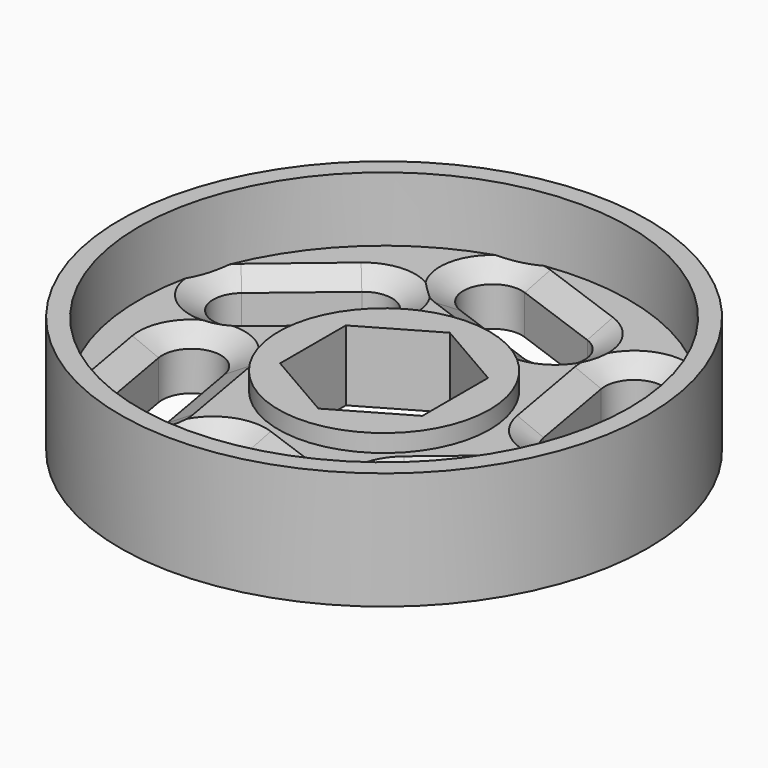
from build123d import *

# Parameters (mm, degrees)
F1_START     = 2
F0_R         = 20.9
F0_R_2       = 9
F1_DEPTH     = 4.5
F2_START     = 2
F0_R_3       = 8
F2_DEPTH     = 6
F3_START     = 2
F3_DEPTH     = 6
F4_START     = 2
F0_R_4       = 22.5
F4_DEPTH     = 10
F5_T1_DEPTH  = 8
F5_T3_DEPTH  = 8
F5_T5_DEPTH  = 8
F5_T7_DEPTH  = 8
F5_T9_DEPTH  = 8
F5_T11_DEPTH = 8
F5_T13_DEPTH = 8
F5_T15_DEPTH = 8
F5_T17_DEPTH = 8
F5_T19_DEPTH = 8
F5_T21_DEPTH = 8
F5_T23_DEPTH = 8
F5_T26_ANGLE = 180
F5_T30_ANGLE = 180
F5_S31_R     = 20.9
F5_T32_DEPTH = 7
F5_T34_ANGLE = 180
F5_T38_ANGLE = 180
F5_S39_R     = 20.9
F5_T40_DEPTH = 7
F5_T44_ANGLE = 180
F5_S45_R     = 20.9
F5_T46_DEPTH = 7
F5_T48_ANGLE = 180
F5_T52_ANGLE = 180
F5_S53_R     = 20.9
F5_T54_DEPTH = 7
F5_T56_ANGLE = 180
F5_T60_ANGLE = 180
F5_S61_R     = 20.9
F5_T62_DEPTH = 7
F5_T64_ANGLE = 180
F5_T66_ANGLE = 180
F5_T70_ANGLE = 180
F5_S71_R     = 20.9
F5_T72_DEPTH = 7


# Not quite as in the source:
# - a fillet or chamfer that OpenCascade refuses, or shapes differently, is made with other operations: its cross-section is extruded or revolved along the edge and cut away or added
# - a feature names something its author has since deleted; it is built from what else it names


with BuildPart() as f1:
    # F0 (on Top) → F1 (new body)
    with BuildSketch(Plane.XY.offset(F1_START)):
        Circle(F0_R)
        with BuildLine():
            ThreePointArc((4.6138208415, -13.9188490213), (6.1080020351, -17.1231309316), (2.9037201248, -18.6173121253))
            Line((2.9037201248, -18.6173121253), (-4.6138208415, -15.8811509787))
            ThreePointArc((-4.6138208415, -15.8811509787), (-6.1080020351, -12.6768690684), (-2.9037201248, -11.1826878747))
            Line((-2.9037201248, -11.1826878747), (4.6138208415, -13.9188490213))
        make_face(mode=Mode.SUBTRACT)
        with BuildLine():
            ThreePointArc((-9.7471664232, -10.9551105679), (-11.7750653616, -13.8512503946), (-14.6712051883, -11.8233514562))
            Line((-14.6712051883, -11.8233514562), (-16.0603906096, -3.9448894321))
            ThreePointArc((-16.0603906096, -3.9448894321), (-14.0324916712, -1.0487496054), (-11.1363518445, -3.0766485438))
            Line((-11.1363518445, -3.0766485438), (-9.7471664232, -10.9551105679))
        make_face(mode=Mode.SUBTRACT)
        with BuildLine():
            ThreePointArc((14.3609872646, -2.9637384535), (17.8830673967, -3.271880537), (17.5749253131, -6.7939606691))
            Line((17.5749253131, -6.7939606691), (11.4465697681, -11.9362615465))
            ThreePointArc((11.4465697681, -11.9362615465), (7.9244896361, -11.628119463), (8.2326317197, -8.1060393309))
            Line((8.2326317197, -8.1060393309), (14.3609872646, -2.9637384535))
        make_face(mode=Mode.SUBTRACT)
        with BuildLine():
            ThreePointArc((-14.3609872646, 2.9637384535), (-17.8830673967, 3.271880537), (-17.5749253131, 6.7939606691))
            Line((-17.5749253131, 6.7939606691), (-11.4465697681, 11.9362615465))
            ThreePointArc((-11.4465697681, 11.9362615465), (-7.9244896361, 11.628119463), (-8.2326317197, 8.1060393309))
            Line((-8.2326317197, 8.1060393309), (-14.3609872646, 2.9637384535))
        make_face(mode=Mode.SUBTRACT)
        Circle(F0_R_2, mode=Mode.SUBTRACT)
        with BuildLine():
            ThreePointArc((9.7471664232, 10.9551105679), (11.7750653616, 13.8512503946), (14.6712051883, 11.8233514562))
            Line((14.6712051883, 11.8233514562), (16.0603906096, 3.9448894321))
            ThreePointArc((16.0603906096, 3.9448894321), (14.0324916712, 1.0487496054), (11.1363518445, 3.0766485438))
            Line((11.1363518445, 3.0766485438), (9.7471664232, 10.9551105679))
        make_face(mode=Mode.SUBTRACT)
        with BuildLine():
            ThreePointArc((-4.6138208415, 13.9188490213), (-6.1080020351, 17.1231309316), (-2.9037201248, 18.6173121253))
            Line((-2.9037201248, 18.6173121253), (4.6138208415, 15.8811509787))
            ThreePointArc((4.6138208415, 15.8811509787), (6.1080020351, 12.6768690684), (2.9037201248, 11.1826878747))
            Line((2.9037201248, 11.1826878747), (-4.6138208415, 13.9188490213))
        make_face(mode=Mode.SUBTRACT)
    extrude(amount=F1_DEPTH)

    # F0 (on Top) → F2 (join)
    with BuildSketch(Plane.XY.offset(F2_START)):
        Circle(F0_R_2)
        Circle(F0_R_3, mode=Mode.SUBTRACT)
    extrude(amount=F2_DEPTH)

    # F0 (on Top) → F3 (join)
    with BuildSketch(Plane.XY.offset(F3_START)):
        Circle(F0_R_3)
        with BuildLine():
            ThreePointArc((6.0621778265, 3.5), (6.761480784, 1.8117333157), (7, 0))
            ThreePointArc((7, 0), (6.761480784, -1.8117333157), (6.0621778265, -3.5))
            ThreePointArc((6.0621778265, -3.5), (3.5, -6.0621778265), (0, -7))
            ThreePointArc((0, -7), (-3.5, -6.0621778265), (-6.0621778265, -3.5))
            ThreePointArc((-6.0621778265, -3.5), (-7, 0), (-6.0621778265, 3.5))
            ThreePointArc((-6.0621778265, 3.5), (-3.5, 6.0621778265), (0, 7))
            ThreePointArc((0, 7), (3.5, 6.0621778265), (6.0621778265, 3.5))
        make_face(mode=Mode.SUBTRACT)
        with BuildLine():
            Line((-6.0621778265, -3.5), (-6.0621778265, 3.5))
            ThreePointArc((-6.0621778265, 3.5), (-7, 0), (-6.0621778265, -3.5))
        make_face()
        with BuildLine():
            Line((-6.0621778265, 3.5), (0, 7))
            ThreePointArc((0, 7), (-3.5, 6.0621778265), (-6.0621778265, 3.5))
        make_face()
        with BuildLine():
            Line((0, 7), (6.0621778265, 3.5))
            ThreePointArc((6.0621778265, 3.5), (3.5, 6.0621778265), (0, 7))
        make_face()
        with BuildLine():
            ThreePointArc((6.0621778265, -3.5), (6.761480784, -1.8117333157), (7, 0))
            ThreePointArc((7, 0), (6.761480784, 1.8117333157), (6.0621778265, 3.5))
            Line((6.0621778265, 3.5), (6.0621778265, -3.5))
        make_face()
        with BuildLine():
            ThreePointArc((0, -7), (3.5, -6.0621778265), (6.0621778265, -3.5))
            Line((6.0621778265, -3.5), (0, -7))
        make_face()
        with BuildLine():
            ThreePointArc((-6.0621778265, -3.5), (-3.5, -6.0621778265), (0, -7))
            Line((0, -7), (-6.0621778265, -3.5))
        make_face()
    extrude(amount=F3_DEPTH)

    # F0 (on Top) → F4 (join)
    with BuildSketch(Plane.XY.offset(F4_START)):
        Circle(F0_R_4)
        Circle(F0_R, mode=Mode.SUBTRACT)
    extrude(amount=F4_DEPTH)

    # F5: chamfer of 2 x 1.1547005384 on 24 edges, made by hand

    # F5_s2 → F5_t1 (cut)
    with BuildSketch(Plane(origin=(1.029997209, -0.3748883255, 0), x_dir=(0, 0, 1), z_dir=(0.9396926208, -0.3420201433, 0))):
        Polygon((5.3452994616, 11.5014200497), (6.5, 9.5014200497), (6.5, 11.5014200497), align=None)
    extrude(amount=F5_T1_DEPTH, mode=Mode.SUBTRACT)

    # F5_s4 → F5_t3 (cut)
    with BuildSketch(Plane(origin=(-1.029997209, 0.3748883255, 0), x_dir=(0, 0, 1), z_dir=(-0.9396926208, 0.3420201433, 0))):
        Polygon((5.3452994616, 11.5014200497), (6.5, 9.5014200497), (6.5, 11.5014200497), align=None)
    extrude(amount=F5_T3_DEPTH, mode=Mode.SUBTRACT)

    # F5_s6 → F5_t5 (cut)
    with BuildSketch(Plane(origin=(-0.1903357911, 1.0794479116, 0), x_dir=(0, 0, 1), z_dir=(-0.1736481777, 0.984807753, 0))):
        Polygon((5.3452994616, 11.5014200497), (6.5, 9.5014200497), (6.5, 11.5014200497), align=None)
    extrude(amount=F5_T5_DEPTH, mode=Mode.SUBTRACT)

    # F5_s8 → F5_t7 (cut)
    with BuildSketch(Plane(origin=(0.8396614179, 0.7045595861, 0), x_dir=(0, 0, 1), z_dir=(0.7660444431, 0.6427876097, 0))):
        Polygon((5.3452994616, 11.5014200497), (6.5, 9.5014200497), (6.5, 11.5014200497), align=None)
    extrude(amount=F5_T7_DEPTH, mode=Mode.SUBTRACT)

    # F5_s10 → F5_t9 (cut)
    with BuildSketch(Plane(origin=(-0.8396614179, -0.7045595861, 0), x_dir=(0, 0, 1), z_dir=(-0.7660444431, -0.6427876097, 0))):
        Polygon((5.3452994616, 11.5014200497), (6.5, 9.5014200497), (6.5, 11.5014200497), align=None)
    extrude(amount=F5_T9_DEPTH, mode=Mode.SUBTRACT)

    # F5_s12 → F5_t11 (cut)
    with BuildSketch(Plane(origin=(0.1903357911, -1.0794479116, 0), x_dir=(0, 0, 1), z_dir=(0.1736481777, -0.984807753, 0))):
        Polygon((5.3452994616, 11.5014200497), (6.5, 9.5014200497), (6.5, 11.5014200497), align=None)
    extrude(amount=F5_T11_DEPTH, mode=Mode.SUBTRACT)

    # F5_s14 → F5_t13 (cut)
    with BuildSketch(Plane(origin=(8.5475381753, -3.1110494721, 0), x_dir=(0, 0, 1), z_dir=(-0.9396926208, 0.3420201433, 0))):
        Polygon((5.3452994616, -16.5014200497), (6.5, -18.5014200497), (6.5, -16.5014200497), align=None)
    extrude(amount=F5_T13_DEPTH, mode=Mode.SUBTRACT)

    # F5_s16 → F5_t15 (cut)
    with BuildSketch(Plane(origin=(1.5795212124, -8.9579099357, 0), x_dir=(0, 0, 1), z_dir=(-0.1736481777, 0.984807753, 0))):
        Polygon((5.3452994616, -16.5014200497), (6.5, -18.5014200497), (6.5, -16.5014200497), align=None)
    extrude(amount=F5_T15_DEPTH, mode=Mode.SUBTRACT)

    # F5_s18 → F5_t17 (cut)
    with BuildSketch(Plane(origin=(6.9680169629, 5.8468604636, 0), x_dir=(0, 0, 1), z_dir=(-0.7660444431, -0.6427876097, 0))):
        Polygon((5.3452994616, -16.5014200497), (6.5, -18.5014200497), (6.5, -16.5014200497), align=None)
    extrude(amount=F5_T17_DEPTH, mode=Mode.SUBTRACT)

    # F5_s20 → F5_t19 (cut)
    with BuildSketch(Plane(origin=(-6.9680169629, -5.8468604636, 0), x_dir=(0, 0, 1), z_dir=(0.7660444431, 0.6427876097, 0))):
        Polygon((5.3452994616, -16.5014200497), (6.5, -18.5014200497), (6.5, -16.5014200497), align=None)
    extrude(amount=F5_T19_DEPTH, mode=Mode.SUBTRACT)

    # F5_s22 → F5_t21 (cut)
    with BuildSketch(Plane(origin=(-1.5795212124, 8.9579099357, 0), x_dir=(0, 0, 1), z_dir=(0.1736481777, -0.984807753, 0))):
        Polygon((5.3452994616, -16.5014200497), (6.5, -18.5014200497), (6.5, -16.5014200497), align=None)
    extrude(amount=F5_T21_DEPTH, mode=Mode.SUBTRACT)

    # F5_s24 → F5_t23 (cut)
    with BuildSketch(Plane(origin=(-8.5475381753, 3.1110494721, 0), x_dir=(0, 0, 1), z_dir=(0.9396926208, -0.3420201433, 0))):
        Polygon((5.3452994616, -16.5014200497), (6.5, -18.5014200497), (6.5, -16.5014200497), align=None)
    extrude(amount=F5_T23_DEPTH, mode=Mode.SUBTRACT)

    # F5_s25 → F5_t26 (revolve, cut)
    with BuildSketch(Plane(origin=(1.029997209, -0.3748883255, 0), x_dir=(0, 0, 1), z_dir=(0.9396926208, -0.3420201433, 0))):
        Polygon((5.3452994616, 16.5014200497), (6.5, 18.5014200497), (6.5, 16.5014200497), align=None)
    revolve(axis=Axis((-3.7587704831, -13.5319194267, 6.5), (0, 0, -1)), revolution_arc=F5_T26_ANGLE, mode=Mode.SUBTRACT)


with BuildPart() as f5_tool28:
    # F5_s29 → F5_t30 (revolve)
    with BuildSketch(Plane(origin=(8.5475381753, -3.1110494721, 0), x_dir=(0, 0, 1), z_dir=(-0.9396926208, 0.3420201433, 0))):
        Polygon((5.3452994616, -11.5014200497), (6.5, -9.5014200497), (6.5, -11.5014200497), align=None)
    revolve(axis=Axis((3.7587704831, -16.2680805733, 6.5), (0, 0, -1)), revolution_arc=F5_T30_ANGLE)

    # F5_s31 → F5_t32 (intersect, symmetric)
    with BuildSketch(Plane.XY.offset(5.9)):
        Circle(F5_S31_R)
    extrude(amount=F5_T32_DEPTH, both=True, mode=Mode.INTERSECT)


with BuildPart() as f1_1:
    add(f1.part)

    # F5_t27: cut F5_tool28
    add(f5_tool28.part, mode=Mode.SUBTRACT)

    # F5_s33 → F5_t34 (revolve, cut)
    with BuildSketch(Plane(origin=(0.1903357911, -1.0794479116, 0), x_dir=(0, 0, 1), z_dir=(0.1736481777, -0.984807753, 0))):
        Polygon((5.3452994616, 16.5014200497), (6.5, 18.5014200497), (6.5, 16.5014200497), align=None)
    revolve(axis=Axis((-13.5983712271, -3.510768988, 6.5), (0, 0, -1)), revolution_arc=F5_T34_ANGLE, mode=Mode.SUBTRACT)


with BuildPart() as f5_tool36:
    # F5_s37 → F5_t38 (revolve)
    with BuildSketch(Plane(origin=(1.5795212124, -8.9579099357, 0), x_dir=(0, 0, 1), z_dir=(-0.1736481777, 0.984807753, 0))):
        Polygon((5.3452994616, -11.5014200497), (6.5, -9.5014200497), (6.5, -11.5014200497), align=None)
    revolve(axis=Axis((-12.2091858057, -11.389231012, 6.5), (0, 0, -1)), revolution_arc=F5_T38_ANGLE)

    # F5_s39 → F5_t40 (intersect, symmetric)
    with BuildSketch(Plane.XY.offset(5.9)):
        Circle(F5_S39_R)
    extrude(amount=F5_T40_DEPTH, both=True, mode=Mode.INTERSECT)


with BuildPart() as f1_2:
    add(f1_1.part)

    # F5_t35: cut F5_tool36
    add(f5_tool36.part, mode=Mode.SUBTRACT)


with BuildPart() as f5_tool42:
    # F5_s43 → F5_t44 (revolve)
    with BuildSketch(Plane(origin=(6.9680169629, 5.8468604636, 0), x_dir=(0, 0, 1), z_dir=(-0.7660444431, -0.6427876097, 0))):
        Polygon((5.3452994616, -11.5014200497), (6.5, -9.5014200497), (6.5, -11.5014200497), align=None)
    revolve(axis=Axis((15.9679562889, -4.8788495613, 6.5), (0, 0, -1)), revolution_arc=F5_T44_ANGLE)

    # F5_s45 → F5_t46 (intersect, symmetric)
    with BuildSketch(Plane.XY.offset(5.9)):
        Circle(F5_S45_R)
    extrude(amount=F5_T46_DEPTH, both=True, mode=Mode.INTERSECT)


with BuildPart() as f1_3:
    add(f1_2.part)

    # F5_t41: cut F5_tool42
    add(f5_tool42.part, mode=Mode.SUBTRACT)

    # F5_s47 → F5_t48 (revolve, cut)
    with BuildSketch(Plane(origin=(0.8396614179, 0.7045595861, 0), x_dir=(0, 0, 1), z_dir=(0.7660444431, 0.6427876097, 0))):
        Polygon((5.3452994616, 16.5014200497), (6.5, 18.5014200497), (6.5, 16.5014200497), align=None)
    revolve(axis=Axis((9.8396007439, -10.0211504387, 6.5), (0, 0, -1)), revolution_arc=F5_T48_ANGLE, mode=Mode.SUBTRACT)


with BuildPart() as f5_tool50:
    # F5_s51 → F5_t52 (revolve)
    with BuildSketch(Plane(origin=(-6.9680169629, -5.8468604636, 0), x_dir=(0, 0, 1), z_dir=(0.7660444431, 0.6427876097, 0))):
        Polygon((5.3452994616, -11.5014200497), (6.5, -9.5014200497), (6.5, -11.5014200497), align=None)
    revolve(axis=Axis((-15.9679562889, 4.8788495613, 6.5), (0, 0, -1)), revolution_arc=F5_T52_ANGLE)

    # F5_s53 → F5_t54 (intersect, symmetric)
    with BuildSketch(Plane.XY.offset(5.9)):
        Circle(F5_S53_R)
    extrude(amount=F5_T54_DEPTH, both=True, mode=Mode.INTERSECT)


with BuildPart() as f1_4:
    add(f1_3.part)

    # F5_t49: cut F5_tool50
    add(f5_tool50.part, mode=Mode.SUBTRACT)

    # F5_s55 → F5_t56 (revolve, cut)
    with BuildSketch(Plane(origin=(-0.8396614179, -0.7045595861, 0), x_dir=(0, 0, 1), z_dir=(-0.7660444431, -0.6427876097, 0))):
        Polygon((5.3452994616, 16.5014200497), (6.5, 18.5014200497), (6.5, 16.5014200497), align=None)
    revolve(axis=Axis((-9.8396007439, 10.0211504387, 6.5), (0, 0, -1)), revolution_arc=F5_T56_ANGLE, mode=Mode.SUBTRACT)


with BuildPart() as f5_tool58:
    # F5_s59 → F5_t60 (revolve)
    with BuildSketch(Plane(origin=(-1.5795212124, 8.9579099357, 0), x_dir=(0, 0, 1), z_dir=(0.1736481777, -0.984807753, 0))):
        Polygon((5.3452994616, -11.5014200497), (6.5, -9.5014200497), (6.5, -11.5014200497), align=None)
    revolve(axis=Axis((12.2091858057, 11.389231012, 6.5), (0, 0, -1)), revolution_arc=F5_T60_ANGLE)

    # F5_s61 → F5_t62 (intersect, symmetric)
    with BuildSketch(Plane.XY.offset(5.9)):
        Circle(F5_S61_R)
    extrude(amount=F5_T62_DEPTH, both=True, mode=Mode.INTERSECT)


with BuildPart() as f1_5:
    add(f1_4.part)

    # F5_t57: cut F5_tool58
    add(f5_tool58.part, mode=Mode.SUBTRACT)

    # F5_s63 → F5_t64 (revolve, cut)
    with BuildSketch(Plane(origin=(-0.1903357911, 1.0794479116, 0), x_dir=(0, 0, 1), z_dir=(-0.1736481777, 0.984807753, 0))):
        Polygon((5.3452994616, 16.5014200497), (6.5, 18.5014200497), (6.5, 16.5014200497), align=None)
    revolve(axis=Axis((13.5983712271, 3.510768988, 6.5), (0, 0, -1)), revolution_arc=F5_T64_ANGLE, mode=Mode.SUBTRACT)

    # F5_s65 → F5_t66 (revolve, cut)
    with BuildSketch(Plane(origin=(-1.029997209, 0.3748883255, 0), x_dir=(0, 0, 1), z_dir=(-0.9396926208, 0.3420201433, 0))):
        Polygon((5.3452994616, 16.5014200497), (6.5, 18.5014200497), (6.5, 16.5014200497), align=None)
    revolve(axis=Axis((3.7587704831, 13.5319194267, 6.5), (0, 0, -1)), revolution_arc=F5_T66_ANGLE, mode=Mode.SUBTRACT)


with BuildPart() as f5_tool68:
    # F5_s69 → F5_t70 (revolve)
    with BuildSketch(Plane(origin=(-8.5475381753, 3.1110494721, 0), x_dir=(0, 0, 1), z_dir=(0.9396926208, -0.3420201433, 0))):
        Polygon((5.3452994616, -11.5014200497), (6.5, -9.5014200497), (6.5, -11.5014200497), align=None)
    revolve(axis=Axis((-3.7587704831, 16.2680805733, 6.5), (0, 0, -1)), revolution_arc=F5_T70_ANGLE)

    # F5_s71 → F5_t72 (intersect, symmetric)
    with BuildSketch(Plane.XY.offset(5.9)):
        Circle(F5_S71_R)
    extrude(amount=F5_T72_DEPTH, both=True, mode=Mode.INTERSECT)


with BuildPart() as f1_6:
    add(f1_5.part)

    # F5_t67: cut F5_tool68
    add(f5_tool68.part, mode=Mode.SUBTRACT)


solid = f1_6.part
